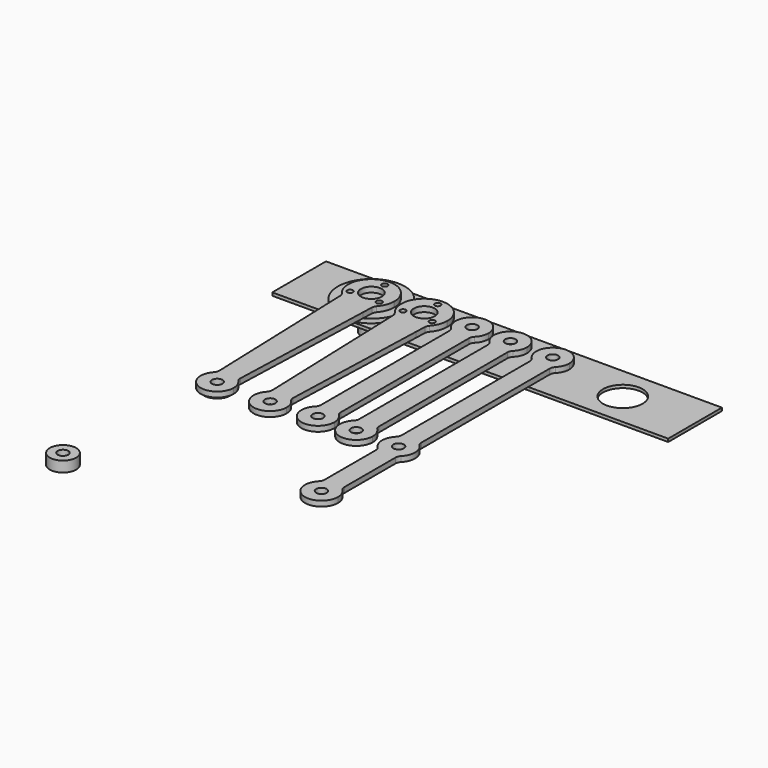
from build123d import *

# Parameters (mm, degrees)
F0_R      = 25.4
F0_R_2    = 7.93
F0_R_3    = 3.99
F1_DEPTH  = 3.17
F2_DEPTH  = 18.85
F3_R      = 7.93
F4_DEPTH  = 4
F5_R      = 5
F6_R      = 4
F7_DEPTH  = 26.021
F8_R      = 10
F8_R_2    = 4
F9_DEPTH  = 2
F10_W     = 300
F10_H     = 50.9
F10_R     = 25.4
F10_R_2   = 15
F11_DEPTH = 2.29
F12_R     = 4
F13_DEPTH = 4
F14_R     = 5
F15_R     = 10
F15_R_2   = 4
F16_DEPTH = 8
F17_D     = 4.318
F17_2_D   = 4.318
F18_R     = 4
F19_DEPTH = 4
F20_R     = 5


# Not quite as in the source:
# - a feature names something its author has since deleted; it is built from what else it names


with BuildPart() as f1:
    # F0 (on Top) → F1 (new body)
    with BuildSketch(Plane.XY):
        Circle(F0_R)
        Circle(F0_R_2, mode=Mode.SUBTRACT)
        Circle(F0_R_2)
        Circle(F0_R_3, mode=Mode.SUBTRACT)
        Circle(F0_R_3)
    extrude(amount=F1_DEPTH)

    # F0 (on Top) → F2 (join)
    with BuildSketch(Plane.XY):
        Circle(F0_R_2)
        Circle(F0_R_3, mode=Mode.SUBTRACT)
    extrude(amount=-F2_DEPTH)

    # F17 (through all)
    with Locations(Plane.XY.offset(7.17)):
        with Locations((0, 12.715), (11.0115130091, -6.3575), (-11.0115130091, -6.3575)):
            Hole(F17_D / 2)


with BuildPart() as f4:
    # F3 (on face) → F4 (new body)
    with BuildSketch(Plane.XY.offset(3.17)):
        with BuildLine():
            ThreePointArc((17.5, 0), (-0.3000393289, 17.4974277081), (-17.4897115887, -0.5999904534))
            ThreePointArc((-17.4897115887, -0.5999904534), (-15.9655514533, -7.1659728433), (-12.0727452916, -12.6688129328))
            ThreePointArc((-12.0727452916, -12.6688129328), (0.0004405364, -17.4999999945), (12.0733831132, -12.66820509))
            ThreePointArc((12.0733831132, -12.66820509), (15.9659122126, -7.1651690294), (17.4897417733, -0.5991099265))
            ThreePointArc((17.4897417733, -0.5991099265), (17.4974352554, -0.2995988715), (17.5, 0))
        make_face()
        Circle(F3_R, mode=Mode.SUBTRACT)
        with BuildLine():
            ThreePointArc((12.0733831132, -12.66820509), (0.0004405364, -17.4999999945), (-12.0727452916, -12.6688129328))
            Line((-12.0727452916, -12.6688129328), (-11.7345611681, -22.5268744879))
            ThreePointArc((-11.7345611681, -22.5268744879), (0.0006394071, -25.399999992), (11.7356953142, -22.5262836592))
            Line((11.7356953142, -22.5262836592), (12.0733831132, -12.66820509))
        make_face()
        with BuildLine():
            ThreePointArc((-7.8312866449, -136.307261705), (-11.2725570094, -140.6481985903), (-12.5, -146.05))
            ThreePointArc((-12.5, -146.05), (0, -158.55), (12.5, -146.05))
            ThreePointArc((12.5, -146.05), (11.2744046762, -140.6520560213), (7.8379521284, -136.3126232263))
            ThreePointArc((7.8379521284, -136.3126232263), (0.0042771071, -133.5500007317), (-7.8312866449, -136.307261705))
        make_face()
        with BuildLine():
            ThreePointArc((11.7356953142, -22.5262836592), (0.0006394071, -25.399999992), (-11.7345611681, -22.5268744879))
            Line((-11.7345611681, -22.5268744879), (-7.8312866449, -136.307261705))
            ThreePointArc((-7.8312866449, -136.307261705), (0.0042771071, -133.5500007317), (7.8379521284, -136.3126232263))
            Line((7.8379521284, -136.3126232263), (11.7356953142, -22.5262836592))
        make_face()
    extrude(amount=F4_DEPTH)

    # F5
    f5_edges = [f4.edges().sort_by_distance(p)[0] for p in [
        (-12.072745, -12.668813, 5.17),
        (12.073383, -12.668205, 5.17),
        (-7.831287, -136.307262, 5.17),
        (7.837952, -136.312623, 5.17),
    ]]
    fillet(f5_edges, radius=F5_R)

    # F6 (on face) → F7 (cut, through all)
    with BuildSketch(Plane.XY.offset(7.17)):
        with Locations((0, -146.05)):
            Circle(F6_R)
    extrude(amount=-F7_DEPTH, mode=Mode.SUBTRACT)

    # F17#2 (through all)
    with Locations(Plane.XY.offset(7.17)):
        with Locations((0, 12.715), (11.0115130091, -6.3575), (-11.0115130091, -6.3575)):
            Hole(F17_2_D / 2)


with BuildPart() as f9:
    # F8 (on face) → F9 (new body)
    with BuildSketch(Plane(origin=(0, 0, 3.17), x_dir=(1, 0, 0), z_dir=(0, 0, -1))):
        with Locations((0, 146.05)):
            Circle(F8_R)
        with Locations((0, 146.05)):
            Circle(F8_R_2, mode=Mode.SUBTRACT)
    extrude(amount=F9_DEPTH)


with BuildPart() as f11:
    # F10 (on face) → F11 (new body)
    with BuildSketch(Plane(origin=(0, 0, 0), x_dir=(1, 0, 0), z_dir=(0, 0, -1))):
        with Locations((95.25, 0)):
            Rectangle(F10_W, F10_H)
        Circle(F10_R, mode=Mode.SUBTRACT)
        with Locations((190.5, 0)):
            Circle(F10_R_2, mode=Mode.SUBTRACT)
        Circle(F10_R)
        Circle(F10_R_2, mode=Mode.SUBTRACT)
    extrude(amount=F11_DEPTH)


with BuildPart() as f13:
    # F12 (on face) → F13 (new body)
    with BuildSketch(Plane.XY.offset(7.17)):
        with BuildLine():
            ThreePointArc((-9.2181924514, -137.607552018), (-11.6506953793, -141.5210600381), (-12.5, -146.05))
            ThreePointArc((-12.5, -146.05), (-11.1803398875, -151.6401699437), (-7.5, -156.05))
            ThreePointArc((-7.5, -156.05), (0, -158.55), (7.5, -156.05))
            ThreePointArc((7.5, -156.05), (11.1803398875, -151.6401699437), (12.5, -146.05))
            ThreePointArc((12.5, -146.05), (11.6519392697, -141.5242612476), (9.2228301991, -137.612618705))
            ThreePointArc((9.2228301991, -137.612618705), (0.0034343857, -133.5500004718), (-9.2181924514, -137.607552018))
        make_face()
        with Locations((0, -146.05)):
            Circle(F12_R, mode=Mode.SUBTRACT)
        with BuildLine():
            ThreePointArc((7.5, -156.05), (0, -158.55), (-7.5, -156.05))
            Line((-7.5, -156.05), (-7.5, -282.1))
            ThreePointArc((-7.5, -282.1), (0, -279.6), (7.5, -282.1))
            Line((7.5, -282.1), (7.5, -156.05))
        make_face()
        with BuildLine():
            ThreePointArc((-7.5, -282.1), (-11.1803398875, -286.5098300563), (-12.5, -292.1))
            ThreePointArc((-12.5, -292.1), (0, -304.6), (12.5, -292.1))
            ThreePointArc((12.5, -292.1), (11.1803398875, -286.5098300563), (7.5, -282.1))
            ThreePointArc((7.5, -282.1), (0, -279.6), (-7.5, -282.1))
        make_face()
        with Locations((0, -292.1)):
            Circle(F12_R, mode=Mode.SUBTRACT)
    extrude(amount=F13_DEPTH)

    # F14
    f14_edges = [f13.edges().sort_by_distance(p)[0] for p in [
        (-7.5, -156.05, 9.17),
        (-7.5, -282.1, 9.17),
        (7.5, -156.05, 9.17),
        (7.5, -282.1, 9.17),
    ]]
    fillet(f14_edges, radius=F14_R)


with BuildPart() as f16:
    # F15 (on face) → F16 (new body)
    with BuildSketch(Plane.XY.offset(11.17)):
        with Locations((0, -292.1)):
            Circle(F15_R)
        with Locations((0, -292.1)):
            Circle(F15_R_2, mode=Mode.SUBTRACT)
    extrude(amount=F16_DEPTH)


with BuildPart() as f19:
    # F18 (on face) → F19 (new body)
    with BuildSketch(Plane.XY.offset(11.17)):
        with BuildLine():
            ThreePointArc((69.9232488871, -100.1979651928), (57.4232488871, -87.6979651928), (44.9232488871, -100.1979651928))
            ThreePointArc((44.9232488871, -100.1979651928), (46.2429089996, -105.7881351365), (49.9232488871, -110.1979651928))
            ThreePointArc((49.9232488871, -110.1979651928), (57.4232488871, -112.6979651928), (64.9232488871, -110.1979651928))
            ThreePointArc((64.9232488871, -110.1979651928), (68.6035887746, -105.7881351365), (69.9232488871, -100.1979651928))
        make_face()
        with Locations((57.4232488871, -100.1979651928)):
            Circle(F18_R, mode=Mode.SUBTRACT)
        with BuildLine():
            ThreePointArc((64.9232488871, -110.1979651928), (57.4232488871, -112.6979651928), (49.9232488871, -110.1979651928))
            Line((49.9232488871, -110.1979651928), (49.9232488871, -236.2479651928))
            ThreePointArc((49.9232488871, -236.2479651928), (57.4232488871, -233.7479651928), (64.9232488871, -236.2479651928))
            Line((64.9232488871, -236.2479651928), (64.9232488871, -110.1979651928))
        make_face()
        with BuildLine():
            ThreePointArc((49.9232488871, -236.2479651928), (46.2429089996, -240.657795249), (44.9232488871, -246.2479651928))
            ThreePointArc((44.9232488871, -246.2479651928), (46.2429089996, -251.8381351365), (49.9232488871, -256.2479651928))
            ThreePointArc((49.9232488871, -256.2479651928), (57.4232488871, -258.7479651928), (64.9232488871, -256.2479651928))
            ThreePointArc((64.9232488871, -256.2479651928), (68.6035887746, -251.8381351365), (69.9232488871, -246.2479651928))
            ThreePointArc((69.9232488871, -246.2479651928), (68.6035887746, -240.657795249), (64.9232488871, -236.2479651928))
            ThreePointArc((64.9232488871, -236.2479651928), (57.4232488871, -233.7479651928), (49.9232488871, -236.2479651928))
        make_face()
        with Locations((57.4232488871, -246.2479651928)):
            Circle(F18_R, mode=Mode.SUBTRACT)
        with BuildLine():
            ThreePointArc((64.9232488871, -256.2479651928), (57.4232488871, -258.7479651928), (49.9232488871, -256.2479651928))
            Line((49.9232488871, -256.2479651928), (49.9232488871, -309.2729651928))
            ThreePointArc((49.9232488871, -309.2729651928), (57.4232488871, -306.7729651928), (64.9232488871, -309.2729651928))
            Line((64.9232488871, -309.2729651928), (64.9232488871, -256.2479651928))
        make_face()
        with BuildLine():
            ThreePointArc((64.9232488871, -309.2729651928), (57.4232488871, -306.7729651928), (49.9232488871, -309.2729651928))
            ThreePointArc((49.9232488871, -309.2729651928), (51.8330789433, -330.4533050803), (69.9232488871, -319.2729651928))
            ThreePointArc((69.9232488871, -319.2729651928), (68.6035887746, -313.682795249), (64.9232488871, -309.2729651928))
        make_face()
        with Locations((57.4232488871, -319.2729651928)):
            Circle(F18_R, mode=Mode.SUBTRACT)
    extrude(amount=F19_DEPTH)

    # F20
    f20_edges = [f19.edges().sort_by_distance(p)[0] for p in [
        (49.923249, -110.197965, 13.17),
        (64.923249, -110.197965, 13.17),
        (64.923249, -236.247965, 13.17),
        (64.923249, -256.247965, 13.17),
        (64.923249, -309.272965, 13.17),
        (49.923249, -309.272965, 13.17),
        (49.923249, -256.247965, 13.17),
        (49.923249, -236.247965, 13.17),
    ]]
    fillet(f20_edges, radius=F20_R)


with BuildPart() as f21_1:
    # F21: copy of F4
    add(f4.part.moved(Location((40.1, 0, 0))))


with BuildPart() as f13_1:
    # F22: moved
    add(f13.part.moved(Location((74, 149, -4))))


with BuildPart() as f19_1:
    # F23: moved
    add(f19.part.moved(Location((78.1, 102.6, -8))))


with BuildPart() as f24_1:
    # F24: copy of F13
    add(f13_1.part.moved(Location((29, 0, 0))))


solid = Compound([f1.part, f4.part, f9.part, f11.part, f16.part, f21_1.part, f13_1.part, f19_1.part, f24_1.part])
